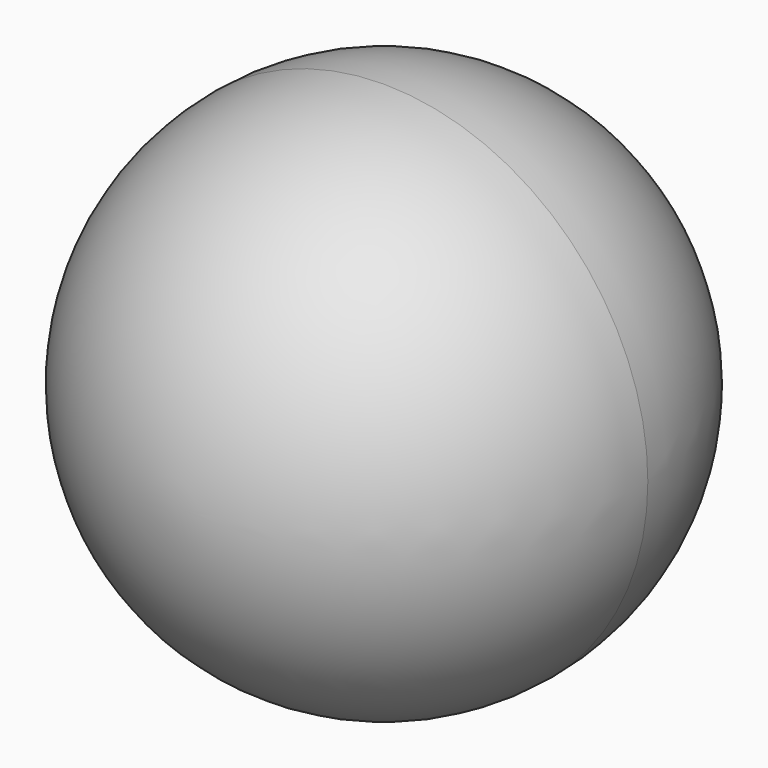
from build123d import *


with BuildPart() as f1:
    # F0 (on Top) → F1 (revolve)
    with BuildSketch(Plane.XY):
        with BuildLine():
            ThreePointArc((0, -19.431), (13.7397918652, -13.7397918652), (19.431, 0))
            ThreePointArc((19.431, 0), (13.7397918652, 13.7397918652), (0, 19.431))
            Line((0, 19.431), (0, 0))
            Line((0, 0), (0, -19.431))
        make_face()
    revolve(axis=Axis((0, 0, 0), (0, -1, 0)))


solid = f1.part
